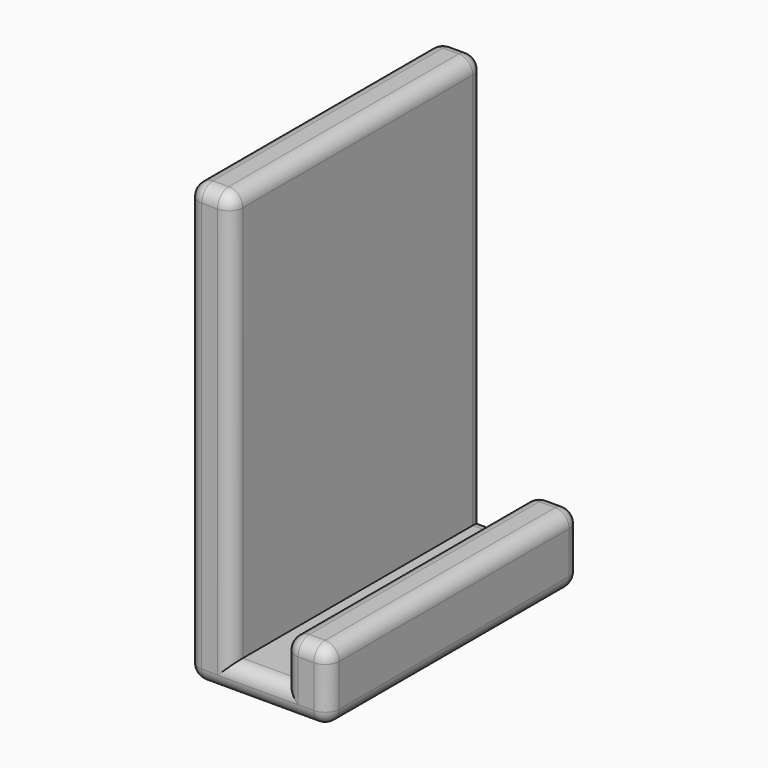
from build123d import *

# Parameters (mm, degrees)
F0_W          = 2.5
F0_H          = 1.5716314532
F0_W_2        = 3
F0_H_2        = 23.4283685468
F0_H_3        = 2.4283685468
F1_DEPTH      = 18
F2_T1_DEPTH   = 16.4
F2_T3_DEPTH   = 22.6283685468
F2_T5_DEPTH   = 3
F2_T7_DEPTH   = 1.6283685468
F2_T9_DEPTH   = 0.9
F2_T11_DEPTH  = 2.4
F2_T13_DEPTH  = 6.4
F2_T15_DEPTH  = 23.4
F2_T17_DEPTH  = 0.9
F2_S21_W      = 0.8
F2_S21_H      = 0.8
F2_T22_DEPTH  = 0.8
F2_S27_W      = 0.8
F2_S27_H      = 0.8
F2_T28_DEPTH  = 0.8
F2_S33_W      = 0.8
F2_S33_H      = 0.8
F2_T34_DEPTH  = 0.8
F2_S39_W      = 0.8
F2_S39_H      = 0.8
F2_T40_DEPTH  = 0.8
F2_S45_W      = 0.8
F2_S45_H      = 0.8
F2_T46_DEPTH  = 0.8
F2_S51_W      = 0.8
F2_S51_H      = 0.8
F2_T52_DEPTH  = 0.8
F2_S57_W      = 0.8
F2_S57_H      = 0.8
F2_T58_DEPTH  = 0.8
F2_S63_W      = 0.8
F2_S63_H      = 0.8
F2_T64_DEPTH  = 0.8
F2_S69_W      = 0.8
F2_S69_H      = 0.8
F2_T70_DEPTH  = 0.8
F2_S75_W      = 0.8
F2_S75_H      = 0.8
F2_T76_DEPTH  = 0.8
F2_S81_W      = 0.8
F2_S81_H      = 0.8
F2_T82_DEPTH  = 0.8
F2_S87_W      = 0.8
F2_S87_H      = 0.8
F2_T88_DEPTH  = 0.8
F2_T95_DEPTH  = 5
F2_T99_DEPTH  = 24.6283685468
F2_T106_DEPTH = 3.6283685468
F2_T110_DEPTH = 5
F2_T117_DEPTH = 3.6283685468
F2_T121_DEPTH = 5
F2_T128_DEPTH = 5
F2_T132_DEPTH = 24.6283685468


# Not quite as in the source:
# - a fillet or chamfer that OpenCascade refuses, or shapes differently, is made with other operations: its cross-section is extruded or revolved along the edge and cut away or added


with BuildPart() as f1:
    # F0 (on Front) → F1 (new body)
    with BuildSketch(Plane.XZ):
        with Locations((1.25, 0.7858157266)):
            Rectangle(F0_W, F0_H)
        with Locations((4, 0.7858157266)):
            Rectangle(F0_W_2, F0_H)
        with Locations((1.25, 13.2858157266)):
            Rectangle(F0_W, F0_H_2)
        with Locations((6.75, 0.7858157266)):
            Rectangle(F0_W, F0_H)
        with Locations((6.75, 2.7858157266)):
            Rectangle(F0_W, F0_H_3)
    extrude(amount=F1_DEPTH)

    # F2: fillet of radius 0.8 on 22 edges, made by hand

    # F2_s2 → F2_t1 (cut)
    with BuildSketch(Plane.XZ.offset(0.8)):
        with BuildLine():
            ThreePointArc((8, 3.2), (7.7656854249, 3.7656854249), (7.2, 4))
            Line((7.2, 4), (8, 4))
            Line((8, 4), (8, 3.2))
        make_face()
        with BuildLine():
            ThreePointArc((7.2, 0), (7.7656854249, 0.2343145751), (8, 0.8))
            Line((8, 0.8), (8, 0))
            Line((8, 0), (7.2, 0))
        make_face()
        with BuildLine():
            ThreePointArc((6.3, 4), (5.7343145751, 3.7656854249), (5.5, 3.2))
            Line((5.5, 3.2), (5.5, 4))
            Line((5.5, 4), (6.3, 4))
        make_face()
        with BuildLine():
            ThreePointArc((2.5, 24.2), (2.2656854249, 24.7656854249), (1.7, 25))
            Line((1.7, 25), (2.5, 25))
            Line((2.5, 25), (2.5, 24.2))
        make_face()
        with BuildLine():
            ThreePointArc((0.8, 25), (0.2343145751, 24.7656854249), (0, 24.2))
            Line((0, 24.2), (0, 25))
            Line((0, 25), (0.8, 25))
        make_face()
        with BuildLine():
            ThreePointArc((0.8, 0), (0.2343145751, 0.2343145751), (0, 0.8))
            Line((0, 0.8), (0, 0))
            Line((0, 0), (0.8, 0))
        make_face()
    extrude(amount=F2_T1_DEPTH, mode=Mode.SUBTRACT)

    # F2_s4 → F2_t3 (cut)
    with BuildSketch(Plane.XY.offset(1.5716314532)):
        with BuildLine():
            ThreePointArc((2.5, -17.2), (2.2656854249, -17.7656854249), (1.7, -18))
            Line((1.7, -18), (2.5, -18))
            Line((2.5, -18), (2.5, -17.2))
        make_face()
        with BuildLine():
            ThreePointArc((2.5, -0.8), (2.2656854249, -0.2343145751), (1.7, 0))
            Line((1.7, 0), (2.5, 0))
            Line((2.5, 0), (2.5, -0.8))
        make_face()
    extrude(amount=F2_T3_DEPTH, mode=Mode.SUBTRACT)

    # F2_s6 → F2_t5 (cut)
    with BuildSketch(Plane.YZ.offset(2.5)):
        with BuildLine():
            ThreePointArc((-17.2, 1.5716314532), (-17.7656854249, 1.3373168782), (-18, 0.7716314532))
            Line((-18, 0.7716314532), (-18, 1.5716314532))
            Line((-18, 1.5716314532), (-17.2, 1.5716314532))
        make_face()
        with BuildLine():
            ThreePointArc((-0.8, 1.5716314532), (-0.2343145751, 1.3373168782), (0, 0.7716314532))
            Line((0, 0.7716314532), (0, 1.5716314532))
            Line((0, 1.5716314532), (-0.8, 1.5716314532))
        make_face()
    extrude(amount=F2_T5_DEPTH, mode=Mode.SUBTRACT)

    # F2_s8 → F2_t7 (cut)
    with BuildSketch(Plane.XY.offset(1.5716314532)):
        with BuildLine():
            ThreePointArc((5.5, -17.2), (5.7343145751, -17.7656854249), (6.3, -18))
            Line((6.3, -18), (5.5, -18))
            Line((5.5, -18), (5.5, -17.2))
        make_face()
        with BuildLine():
            ThreePointArc((5.5, -0.8), (5.7343145751, -0.2343145751), (6.3, 0))
            Line((6.3, 0), (5.5, 0))
            Line((5.5, 0), (5.5, -0.8))
        make_face()
    extrude(amount=F2_T7_DEPTH, mode=Mode.SUBTRACT)

    # F2_s10 → F2_t9 (cut)
    with BuildSketch(Plane.YZ.offset(6.3)):
        with BuildLine():
            ThreePointArc((-17.2, 4), (-17.7656854249, 3.7656854249), (-18, 3.2))
            Line((-18, 3.2), (-18, 4))
            Line((-18, 4), (-17.2, 4))
        make_face()
        with BuildLine():
            ThreePointArc((-0.8, 4), (-0.2343145751, 3.7656854249), (0, 3.2))
            Line((0, 3.2), (0, 4))
            Line((0, 4), (-0.8, 4))
        make_face()
    extrude(amount=F2_T9_DEPTH, mode=Mode.SUBTRACT)

    # F2_s12 → F2_t11 (cut)
    with BuildSketch(Plane.XY.offset(0.8)):
        with BuildLine():
            ThreePointArc((8, -17.2), (7.7656854249, -17.7656854249), (7.2, -18))
            Line((7.2, -18), (8, -18))
            Line((8, -18), (8, -17.2))
        make_face()
        with BuildLine():
            ThreePointArc((8, -0.8), (7.7656854249, -0.2343145751), (7.2, 0))
            Line((7.2, 0), (8, 0))
            Line((8, 0), (8, -0.8))
        make_face()
    extrude(amount=F2_T11_DEPTH, mode=Mode.SUBTRACT)

    # F2_s14 → F2_t13 (cut)
    with BuildSketch(Plane.YZ.offset(0.8)):
        with BuildLine():
            ThreePointArc((-17.2, 0), (-17.7656854249, 0.2343145751), (-18, 0.8))
            Line((-18, 0.8), (-18, 0))
            Line((-18, 0), (-17.2, 0))
        make_face()
        with BuildLine():
            ThreePointArc((-0.8, 0), (-0.2343145751, 0.2343145751), (0, 0.8))
            Line((0, 0.8), (0, 0))
            Line((0, 0), (-0.8, 0))
        make_face()
    extrude(amount=F2_T13_DEPTH, mode=Mode.SUBTRACT)

    # F2_s16 → F2_t15 (cut)
    with BuildSketch(Plane.XY.offset(0.8)):
        with BuildLine():
            ThreePointArc((0, -17.2), (0.2343145751, -17.7656854249), (0.8, -18))
            Line((0.8, -18), (0, -18))
            Line((0, -18), (0, -17.2))
        make_face()
        with BuildLine():
            ThreePointArc((0, -0.8), (0.2343145751, -0.2343145751), (0.8, 0))
            Line((0.8, 0), (0, 0))
            Line((0, 0), (0, -0.8))
        make_face()
    extrude(amount=F2_T15_DEPTH, mode=Mode.SUBTRACT)

    # F2_s18 → F2_t17 (cut)
    with BuildSketch(Plane.YZ.offset(0.8)):
        with BuildLine():
            ThreePointArc((-0.8, 25), (-0.2343145751, 24.7656854249), (0, 24.2))
            Line((0, 24.2), (0, 25))
            Line((0, 25), (-0.8, 25))
        make_face()
        with BuildLine():
            ThreePointArc((-17.2, 25), (-17.7656854249, 24.7656854249), (-18, 24.2))
            Line((-18, 24.2), (-18, 25))
            Line((-18, 25), (-17.2, 25))
        make_face()
    extrude(amount=F2_T17_DEPTH, mode=Mode.SUBTRACT)


with BuildPart() as f2_tool20:
    # F2_s21 → F2_t22 (new body)
    with BuildSketch(Plane.XZ.offset(0.8)):
        with Locations((7.6, 3.6)):
            Rectangle(F2_S21_W, F2_S21_H)
    extrude(amount=-F2_T22_DEPTH)

    # F2_s23 → F2_t24 (revolve, cut)
    with BuildSketch(Plane(origin=(7.2, -0.8, 3.2), x_dir=(-0.7071067812, 0, -0.7071067812), z_dir=(0.7071067812, 0, -0.7071067812))):
        with BuildLine():
            ThreePointArc((0, -0.8), (0.8, 0), (0, 0.8))
            Line((0, 0.8), (0, -0.8))
        make_face()
    revolve(axis=Axis((7.2, -0.8, 3.2), (0, 1, 0)), mode=Mode.SUBTRACT)


with BuildPart() as f1_1:
    add(f1.part)

    # F2_t19: cut F2_tool20
    add(f2_tool20.part, mode=Mode.SUBTRACT)


with BuildPart() as f2_tool26:
    # F2_s27 → F2_t28 (new body)
    with BuildSketch(Plane.YZ.offset(7.2)):
        with Locations((-17.6, 3.6)):
            Rectangle(F2_S27_W, F2_S27_H)
    extrude(amount=F2_T28_DEPTH)

    # F2_s29 → F2_t30 (revolve, cut)
    with BuildSketch(Plane(origin=(7.2, -17.2, 3.2), x_dir=(0, 0.7071067812, -0.7071067812), z_dir=(0, -0.7071067812, -0.7071067812))):
        with BuildLine():
            ThreePointArc((0, -0.8), (0.8, 0), (0, 0.8))
            Line((0, 0.8), (0, -0.8))
        make_face()
    revolve(axis=Axis((7.2, -17.2, 3.2), (1, 0, 0)), mode=Mode.SUBTRACT)


with BuildPart() as f1_2:
    add(f1_1.part)

    # F2_t25: cut F2_tool26
    add(f2_tool26.part, mode=Mode.SUBTRACT)


with BuildPart() as f2_tool32:
    # F2_s33 → F2_t34 (new body)
    with BuildSketch(Plane.XZ.offset(17.2)):
        with Locations((2.1, 24.6)):
            Rectangle(F2_S33_W, F2_S33_H)
    extrude(amount=F2_T34_DEPTH)

    # F2_s35 → F2_t36 (revolve, cut)
    with BuildSketch(Plane(origin=(1.7, -17.2, 24.2), x_dir=(-0.7071067812, 0, -0.7071067812), z_dir=(-0.7071067812, 0, 0.7071067812))):
        with BuildLine():
            ThreePointArc((0, -0.8), (0.8, 0), (0, 0.8))
            Line((0, 0.8), (0, -0.8))
        make_face()
    revolve(axis=Axis((1.7, -17.2, 24.2), (0, -1, 0)), mode=Mode.SUBTRACT)


with BuildPart() as f1_3:
    add(f1_2.part)

    # F2_t31: cut F2_tool32
    add(f2_tool32.part, mode=Mode.SUBTRACT)


with BuildPart() as f2_tool38:
    # F2_s39 → F2_t40 (new body)
    with BuildSketch(Plane.XZ.offset(17.2)):
        with Locations((5.9, 3.6)):
            Rectangle(F2_S39_W, F2_S39_H)
    extrude(amount=F2_T40_DEPTH)

    # F2_s41 → F2_t42 (revolve, cut)
    with BuildSketch(Plane(origin=(6.3, -17.2, 3.2), x_dir=(0.7071067812, 0, -0.7071067812), z_dir=(-0.7071067812, 0, -0.7071067812))):
        with BuildLine():
            ThreePointArc((0, -0.8), (0.8, 0), (0, 0.8))
            Line((0, 0.8), (0, -0.8))
        make_face()
    revolve(axis=Axis((6.3, -17.2, 3.2), (0, -1, 0)), mode=Mode.SUBTRACT)


with BuildPart() as f1_4:
    add(f1_3.part)

    # F2_t37: cut F2_tool38
    add(f2_tool38.part, mode=Mode.SUBTRACT)


with BuildPart() as f2_tool44:
    # F2_s45 → F2_t46 (new body)
    with BuildSketch(Plane.XY.offset(0.8)):
        with Locations((7.6, -17.6)):
            Rectangle(F2_S45_W, F2_S45_H)
    extrude(amount=-F2_T46_DEPTH)

    # F2_s47 → F2_t48 (revolve, cut)
    with BuildSketch(Plane(origin=(7.2, -17.2, 0.8), x_dir=(-0.7071067812, 0.7071067812, 0), z_dir=(-0.7071067812, -0.7071067812, 0))):
        with BuildLine():
            ThreePointArc((0, -0.8), (0.8, 0), (0, 0.8))
            Line((0, 0.8), (0, -0.8))
        make_face()
    revolve(axis=Axis((7.2, -17.2, 0.8), (0, 0, -1)), mode=Mode.SUBTRACT)


with BuildPart() as f1_5:
    add(f1_4.part)

    # F2_t43: cut F2_tool44
    add(f2_tool44.part, mode=Mode.SUBTRACT)


with BuildPart() as f2_tool50:
    # F2_s51 → F2_t52 (new body)
    with BuildSketch(Plane.XY.offset(0.8)):
        with Locations((0.4, -17.6)):
            Rectangle(F2_S51_W, F2_S51_H)
    extrude(amount=-F2_T52_DEPTH)

    # F2_s53 → F2_t54 (revolve, cut)
    with BuildSketch(Plane(origin=(0.8, -17.2, 0.8), x_dir=(0.7071067812, 0.7071067812, 0), z_dir=(-0.7071067812, 0.7071067812, 0))):
        with BuildLine():
            ThreePointArc((0, -0.8), (0.8, 0), (0, 0.8))
            Line((0, 0.8), (0, -0.8))
        make_face()
    revolve(axis=Axis((0.8, -17.2, 0.8), (0, 0, -1)), mode=Mode.SUBTRACT)


with BuildPart() as f1_6:
    add(f1_5.part)

    # F2_t49: cut F2_tool50
    add(f2_tool50.part, mode=Mode.SUBTRACT)


with BuildPart() as f2_tool56:
    # F2_s57 → F2_t58 (new body)
    with BuildSketch(Plane.XZ.offset(17.2)):
        with Locations((0.4, 24.6)):
            Rectangle(F2_S57_W, F2_S57_H)
    extrude(amount=F2_T58_DEPTH)

    # F2_s59 → F2_t60 (revolve, cut)
    with BuildSketch(Plane(origin=(0.8, -17.2, 24.2), x_dir=(0.7071067812, 0, -0.7071067812), z_dir=(-0.7071067812, 0, -0.7071067812))):
        with BuildLine():
            ThreePointArc((0, -0.8), (0.8, 0), (0, 0.8))
            Line((0, 0.8), (0, -0.8))
        make_face()
    revolve(axis=Axis((0.8, -17.2, 24.2), (0, -1, 0)), mode=Mode.SUBTRACT)


with BuildPart() as f1_7:
    add(f1_6.part)

    # F2_t55: cut F2_tool56
    add(f2_tool56.part, mode=Mode.SUBTRACT)


with BuildPart() as f2_tool62:
    # F2_s63 → F2_t64 (new body)
    with BuildSketch(Plane.XY.offset(0.8)):
        with Locations((7.6, -0.4)):
            Rectangle(F2_S63_W, F2_S63_H)
    extrude(amount=-F2_T64_DEPTH)

    # F2_s65 → F2_t66 (revolve, cut)
    with BuildSketch(Plane(origin=(7.2, -0.8, 0.8), x_dir=(-0.7071067812, -0.7071067812, 0), z_dir=(0.7071067812, -0.7071067812, 0))):
        with BuildLine():
            ThreePointArc((0, -0.8), (0.8, 0), (0, 0.8))
            Line((0, 0.8), (0, -0.8))
        make_face()
    revolve(axis=Axis((7.2, -0.8, 0.8), (0, 0, -1)), mode=Mode.SUBTRACT)


with BuildPart() as f1_8:
    add(f1_7.part)

    # F2_t61: cut F2_tool62
    add(f2_tool62.part, mode=Mode.SUBTRACT)


with BuildPart() as f2_tool68:
    # F2_s69 → F2_t70 (new body)
    with BuildSketch(Plane.XZ.offset(0.8)):
        with Locations((5.9, 3.6)):
            Rectangle(F2_S69_W, F2_S69_H)
    extrude(amount=-F2_T70_DEPTH)

    # F2_s71 → F2_t72 (revolve, cut)
    with BuildSketch(Plane(origin=(6.3, -0.8, 3.2), x_dir=(0.7071067812, 0, -0.7071067812), z_dir=(0.7071067812, 0, 0.7071067812))):
        with BuildLine():
            ThreePointArc((0, -0.8), (0.8, 0), (0, 0.8))
            Line((0, 0.8), (0, -0.8))
        make_face()
    revolve(axis=Axis((6.3, -0.8, 3.2), (0, 1, 0)), mode=Mode.SUBTRACT)


with BuildPart() as f1_9:
    add(f1_8.part)

    # F2_t67: cut F2_tool68
    add(f2_tool68.part, mode=Mode.SUBTRACT)


with BuildPart() as f2_tool74:
    # F2_s75 → F2_t76 (new body)
    with BuildSketch(Plane.XY.offset(0.8)):
        with Locations((0.4, -0.4)):
            Rectangle(F2_S75_W, F2_S75_H)
    extrude(amount=-F2_T76_DEPTH)

    # F2_s77 → F2_t78 (revolve, cut)
    with BuildSketch(Plane(origin=(0.8, -0.8, 0.8), x_dir=(0.7071067812, -0.7071067812, 0), z_dir=(0.7071067812, 0.7071067812, 0))):
        with BuildLine():
            ThreePointArc((0, -0.8), (0.8, 0), (0, 0.8))
            Line((0, 0.8), (0, -0.8))
        make_face()
    revolve(axis=Axis((0.8, -0.8, 0.8), (0, 0, -1)), mode=Mode.SUBTRACT)


with BuildPart() as f1_10:
    add(f1_9.part)

    # F2_t73: cut F2_tool74
    add(f2_tool74.part, mode=Mode.SUBTRACT)


with BuildPart() as f2_tool80:
    # F2_s81 → F2_t82 (new body)
    with BuildSketch(Plane.XZ.offset(0.8)):
        with Locations((2.1, 24.6)):
            Rectangle(F2_S81_W, F2_S81_H)
    extrude(amount=-F2_T82_DEPTH)

    # F2_s83 → F2_t84 (revolve, cut)
    with BuildSketch(Plane(origin=(1.7, -0.8, 24.2), x_dir=(-0.7071067812, 0, -0.7071067812), z_dir=(0.7071067812, 0, -0.7071067812))):
        with BuildLine():
            ThreePointArc((0, -0.8), (0.8, 0), (0, 0.8))
            Line((0, 0.8), (0, -0.8))
        make_face()
    revolve(axis=Axis((1.7, -0.8, 24.2), (0, 1, 0)), mode=Mode.SUBTRACT)


with BuildPart() as f1_11:
    add(f1_10.part)

    # F2_t79: cut F2_tool80
    add(f2_tool80.part, mode=Mode.SUBTRACT)


with BuildPart() as f2_tool86:
    # F2_s87 → F2_t88 (new body)
    with BuildSketch(Plane.XZ.offset(0.8)):
        with Locations((0.4, 24.6)):
            Rectangle(F2_S87_W, F2_S87_H)
    extrude(amount=-F2_T88_DEPTH)

    # F2_s89 → F2_t90 (revolve, cut)
    with BuildSketch(Plane(origin=(0.8, -0.8, 24.2), x_dir=(0.7071067812, 0, -0.7071067812), z_dir=(0.7071067812, 0, 0.7071067812))):
        with BuildLine():
            ThreePointArc((0, -0.8), (0.8, 0), (0, 0.8))
            Line((0, 0.8), (0, -0.8))
        make_face()
    revolve(axis=Axis((0.8, -0.8, 24.2), (0, 1, 0)), mode=Mode.SUBTRACT)


with BuildPart() as f1_12:
    add(f1_11.part)

    # F2_t85: cut F2_tool86
    add(f2_tool86.part, mode=Mode.SUBTRACT)


with BuildPart() as f2_tool93:
    # F2_s94 → F2_t95 (new body)
    with BuildSketch(Plane.YZ.offset(5.5)):
        with BuildLine():
            ThreePointArc((-17.2, 1.5716314532), (-17.7656854249, 1.3373168782), (-18, 0.7716314532))
            Line((-18, 0.7716314532), (-18, 1.5716314532))
            Line((-18, 1.5716314532), (-17.2, 1.5716314532))
        make_face()
    extrude(amount=-F2_T95_DEPTH)

    split(bisect_by=Plane.YZ.offset(2.5), keep=Keep.BOTTOM)


with BuildPart() as f2_tool97:
    # F2_s98 → F2_t99 (new body)
    with BuildSketch(Plane.XY.offset(-0.4283685468)):
        with BuildLine():
            ThreePointArc((2.5, -17.2), (2.2656854249, -17.7656854249), (1.7, -18))
            Line((1.7, -18), (2.5, -18))
            Line((2.5, -18), (2.5, -17.2))
        make_face()
    extrude(amount=F2_T99_DEPTH)

    split(bisect_by=Plane.XY.offset(1.5716314532), keep=Keep.BOTTOM)


with BuildPart() as f2_tool93_1:
    add(f2_tool93.part)

    # F2_t101: intersect F2_tool97
    add(f2_tool97.part, mode=Mode.INTERSECT)


with BuildPart() as f1_13:
    add(f1_12.part)

    # F2_t91: cut F2_tool93
    add(f2_tool93_1.part, mode=Mode.SUBTRACT)


with BuildPart() as f2_tool104:
    # F2_s105 → F2_t106 (new body)
    with BuildSketch(Plane.XY.offset(3.2)):
        with BuildLine():
            ThreePointArc((5.5, -17.2), (5.7343145751, -17.7656854249), (6.3, -18))
            Line((6.3, -18), (5.5, -18))
            Line((5.5, -18), (5.5, -17.2))
        make_face()
    extrude(amount=-F2_T106_DEPTH)

    split(bisect_by=Plane.XY.offset(1.5716314532), keep=Keep.BOTTOM)


with BuildPart() as f2_tool108:
    # F2_s109 → F2_t110 (new body)
    with BuildSketch(Plane.YZ.offset(7.5)):
        with BuildLine():
            ThreePointArc((-17.2, 1.5716314532), (-17.7656854249, 1.3373168782), (-18, 0.7716314532))
            Line((-18, 0.7716314532), (-18, 1.5716314532))
            Line((-18, 1.5716314532), (-17.2, 1.5716314532))
        make_face()
    extrude(amount=-F2_T110_DEPTH)

    split(bisect_by=Plane.YZ.offset(5.5), keep=Keep.TOP)


with BuildPart() as f2_tool104_1:
    add(f2_tool104.part)

    # F2_t112: intersect F2_tool108
    add(f2_tool108.part, mode=Mode.INTERSECT)


with BuildPart() as f1_14:
    add(f1_13.part)

    # F2_t102: cut F2_tool104
    add(f2_tool104_1.part, mode=Mode.SUBTRACT)


with BuildPart() as f2_tool115:
    # F2_s116 → F2_t117 (new body)
    with BuildSketch(Plane.XY.offset(3.2)):
        with BuildLine():
            ThreePointArc((5.5, -0.8), (5.7343145751, -0.2343145751), (6.3, 0))
            Line((6.3, 0), (5.5, 0))
            Line((5.5, 0), (5.5, -0.8))
        make_face()
    extrude(amount=-F2_T117_DEPTH)

    split(bisect_by=Plane.XY.offset(1.5716314532), keep=Keep.BOTTOM)


with BuildPart() as f2_tool119:
    # F2_s120 → F2_t121 (new body)
    with BuildSketch(Plane.YZ.offset(7.5)):
        with BuildLine():
            ThreePointArc((-0.8, 1.5716314532), (-0.2343145751, 1.3373168782), (0, 0.7716314532))
            Line((0, 0.7716314532), (0, 1.5716314532))
            Line((0, 1.5716314532), (-0.8, 1.5716314532))
        make_face()
    extrude(amount=-F2_T121_DEPTH)

    split(bisect_by=Plane.YZ.offset(5.5), keep=Keep.TOP)


with BuildPart() as f2_tool115_1:
    add(f2_tool115.part)

    # F2_t123: intersect F2_tool119
    add(f2_tool119.part, mode=Mode.INTERSECT)


with BuildPart() as f1_15:
    add(f1_14.part)

    # F2_t113: cut F2_tool115
    add(f2_tool115_1.part, mode=Mode.SUBTRACT)


with BuildPart() as f2_tool126:
    # F2_s127 → F2_t128 (new body)
    with BuildSketch(Plane.YZ.offset(5.5)):
        with BuildLine():
            ThreePointArc((-0.8, 1.5716314532), (-0.2343145751, 1.3373168782), (0, 0.7716314532))
            Line((0, 0.7716314532), (0, 1.5716314532))
            Line((0, 1.5716314532), (-0.8, 1.5716314532))
        make_face()
    extrude(amount=-F2_T128_DEPTH)

    split(bisect_by=Plane.YZ.offset(2.5), keep=Keep.BOTTOM)


with BuildPart() as f2_tool130:
    # F2_s131 → F2_t132 (new body)
    with BuildSketch(Plane.XY.offset(-0.4283685468)):
        with BuildLine():
            ThreePointArc((2.5, -0.8), (2.2656854249, -0.2343145751), (1.7, 0))
            Line((1.7, 0), (2.5, 0))
            Line((2.5, 0), (2.5, -0.8))
        make_face()
    extrude(amount=F2_T132_DEPTH)

    split(bisect_by=Plane.XY.offset(1.5716314532), keep=Keep.BOTTOM)


with BuildPart() as f2_tool126_1:
    add(f2_tool126.part)

    # F2_t134: intersect F2_tool130
    add(f2_tool130.part, mode=Mode.INTERSECT)


with BuildPart() as f1_16:
    add(f1_15.part)

    # F2_t124: cut F2_tool126
    add(f2_tool126_1.part, mode=Mode.SUBTRACT)


solid = f1_16.part
